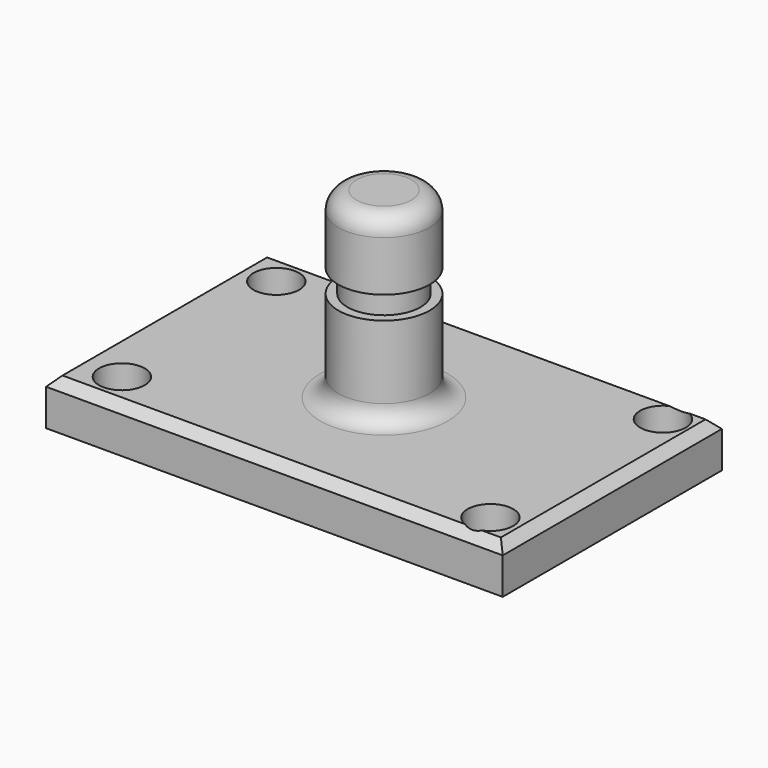
from build123d import *

# Parameters (mm, degrees)
F0_W        = 127
F0_H        = 76.2
F1_DEPTH    = 12.7
F2_R        = 6.35
F3_DEPTH    = 12.701
F4_W        = 12.7
F4_H        = 50.8
F6_W        = 13.0245922636
F6_H        = 6.35
F8_R        = 5.08
F9_T1_DEPTH = 140.0641495789
F9_T3_DEPTH = 89.2641495789


# Not quite as in the source:
# - a fillet or chamfer that OpenCascade refuses, or shapes differently, is made with other operations: its cross-section is extruded or revolved along the edge and cut away or added


with BuildPart() as f1:
    # F0 (on Top) → F1 (new body)
    with BuildSketch(Plane.XY):
        Rectangle(F0_W, F0_H)
    extrude(amount=F1_DEPTH)

    # F2 (on face) → F3 (cut, through all)
    with BuildSketch(Plane.XY.offset(12.7)):
        with Locations((-52.3479245603, 27.9940944165)):
            Circle(F2_R)
        with Locations((53.7015721202, 29.8446007073)):
            Circle(F2_R)
        with Locations((-50.5206361413, -27.9734656215)):
            Circle(F2_R)
        with Locations((53.327344358, -29.6574886888)):
            Circle(F2_R)
    extrude(amount=-F3_DEPTH, mode=Mode.SUBTRACT)

    # F4 (on Front) → F5 (revolve)
    with BuildSketch(Plane.XZ):
        with Locations((6.35, 38.1)):
            Rectangle(F4_W, F4_H)
    revolve(axis=Axis((0, 0, 38.1), (0, 0, 1)))

    # F6 (on Front) → F7 (revolve, cut)
    with BuildSketch(Plane.XZ):
        with Locations((16.6722961318, 41.275)):
            Rectangle(F6_W, F6_H)
    revolve(axis=Axis((0, 0, 38.1), (0, 0, 1)), mode=Mode.SUBTRACT)

    # F8
    f8_edges = [f1.edges().sort_by_distance(p)[0] for p in [
        (-12.7, 0, 63.5),
        (-12.7, 0, 12.7),
    ]]
    fillet(f8_edges, radius=F8_R)

    # F9: chamfer of 2.54 on 4 edges, made by hand

    # F9_s2 → F9_t1 (cut)
    with BuildSketch(Plane.YZ.offset(-70.0320747894)):
        Polygon((-35.56, 12.7), (-38.1, 10.16), (-38.1, 12.7), align=None)
        Polygon((35.56, 12.7), (38.1, 10.16), (38.1, 12.7), align=None)
    extrude(amount=F9_T1_DEPTH, mode=Mode.SUBTRACT)

    # F9_s4 → F9_t3 (cut)
    with BuildSketch(Plane.XZ.offset(-44.6320747894)):
        Polygon((60.96, 12.7), (63.5, 10.16), (63.5, 12.7), align=None)
        Polygon((-60.96, 12.7), (-63.5, 10.16), (-63.5, 12.7), align=None)
    extrude(amount=F9_T3_DEPTH, mode=Mode.SUBTRACT)


solid = f1.part
